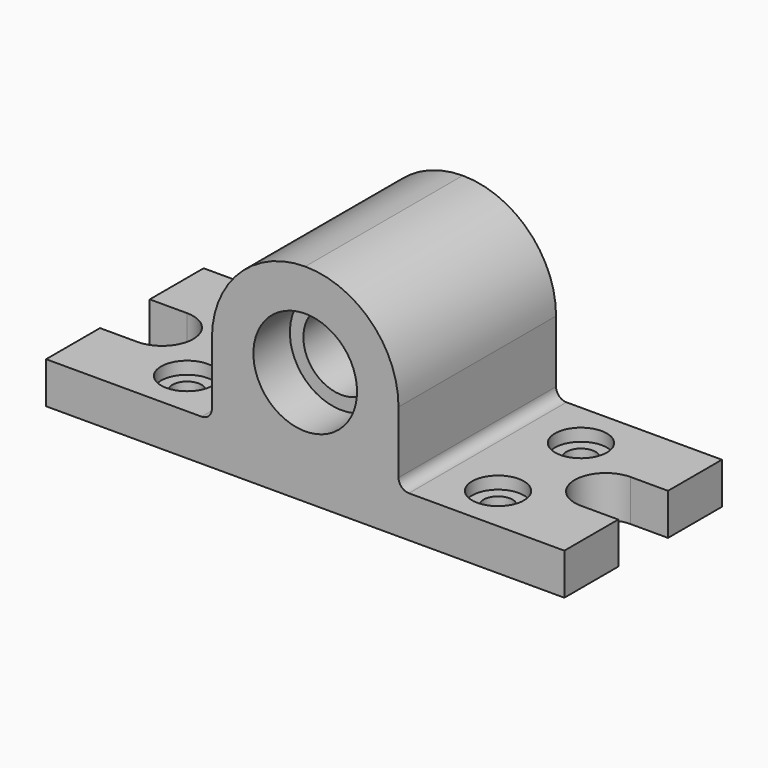
from build123d import *

# Parameters (mm, degrees)
F1_DEPTH  = 47.5
F2_R      = 44.99999
F3_R      = 5
F4_R      = 18.5
F5_DEPTH  = 95.001
F4_R_2    = 25
F6_DEPTH  = 22
F8_DEPTH  = 20.001
F7_R      = 12.5
F7_R_2    = 7
F9_DEPTH  = 6
F10_DEPTH = 20.001


# Not quite as in the source:
# - a fillet or chamfer is up to 0.001 mm smaller than in the source, because OpenCascade refuses the exact size
# - a pattern or mirror of a feature is missing from the dataset's text; its kind, count and spacing are read off the source's solid


with BuildPart() as f1:
    # F0 (on Front) → F1 (new body, symmetric)
    with BuildSketch(Plane.XZ):
        Polygon((-45, 10), (-125, 10), (-125, -10), (125, -10), (125, 10), (45, 10), (45, 90), (-45, 90), align=None)
    extrude(amount=F1_DEPTH, both=True)

    # F2 (radius 45 in the source; OpenCascade refuses exactly that, so slightly less here)
    f2_edges = [f1.edges().sort_by_distance(p)[0] for p in [
        (45, 0, 90),
        (-45, 0, 90),
    ]]
    fillet(f2_edges, radius=F2_R)

    # F3
    f3_edges = [f1.edges().sort_by_distance(p)[0] for p in [
        (45, 0, 10),
        (-45, 0, 10),
    ]]
    fillet(f3_edges, radius=F3_R)

    # F4 (on face) → F5 (cut, through all)
    with BuildSketch(Plane.XZ.offset(47.5)):
        with Locations((0, 45)):
            Circle(F4_R)
    extrude(amount=-F5_DEPTH, mode=Mode.SUBTRACT)

    # F4 (on face) → F6 (cut)
    with BuildSketch(Plane.XZ.offset(47.5)):
        with Locations((0, 45)):
            Circle(F4_R_2)
        with Locations((0, 45)):
            Circle(F4_R, mode=Mode.SUBTRACT)
    extrude(amount=-F6_DEPTH, mode=Mode.SUBTRACT)

    # F7 (on face) → F8 (cut, through all)
    with BuildSketch(Plane.XY.offset(10)):
        with BuildLine():
            Line((125, -15), (125, 15))
            Line((125, 15), (107, 15))
            ThreePointArc((107, 15), (92, 0), (107, -15))
            Line((107, -15), (125, -15))
        make_face()
    f8 = extrude(amount=-F8_DEPTH, mode=Mode.SUBTRACT)

    # F8_copies: F8 across plane
    add(f8.mirror(Plane(origin=(0, 0, 0), x_dir=(0, 0, -1), z_dir=(-1, 0, 0))), mode=Mode.SUBTRACT)

    # F7 (on face) → F9 (cut)
    with BuildSketch(Plane.XY.offset(10)):
        with Locations((75, 25)):
            Circle(F7_R)
        with Locations((75, 25)):
            Circle(F7_R_2, mode=Mode.SUBTRACT)
    f9 = extrude(amount=-F9_DEPTH, mode=Mode.SUBTRACT)

    # F9_copies: F9 across plane
    add(f9.mirror(Plane(origin=(0, 0, 0), x_dir=(0, 0, -1), z_dir=(-1, 0, 0))), mode=Mode.SUBTRACT)

    # F9_copies1: F9 across plane
    add(f9.mirror(Plane(origin=(0, 0, 0), x_dir=(0, 0, -1), z_dir=(0, -1, 0))), mode=Mode.SUBTRACT)

    # F9_copies2: F9 across plane
    add(f9.mirror(Plane(origin=(0, 0, 0), x_dir=(0.316227766, -0.9486832981, 0), z_dir=(-0.9486832981, -0.316227766, 0))), mode=Mode.SUBTRACT)

    # F7 (on face) → F10 (cut, through all)
    with BuildSketch(Plane.XY.offset(10)):
        with Locations((75, 25)):
            Circle(F7_R_2)
    f10 = extrude(amount=-F10_DEPTH, mode=Mode.SUBTRACT)

    # F10_copies: F10 across plane
    add(f10.mirror(Plane(origin=(0, 0, 0), x_dir=(0, 0, -1), z_dir=(0, -1, 0))), mode=Mode.SUBTRACT)

    # F10_copies1: F10 across plane
    add(f10.mirror(Plane(origin=(0, 0, 0), x_dir=(0, 0, -1), z_dir=(-1, 0, 0))), mode=Mode.SUBTRACT)

    # F10_copies2: F10 across plane
    add(f10.mirror(Plane(origin=(0, 0, 0), x_dir=(0.316227766, -0.9486832981, 0), z_dir=(-0.9486832981, -0.316227766, 0))), mode=Mode.SUBTRACT)


solid = f1.part
